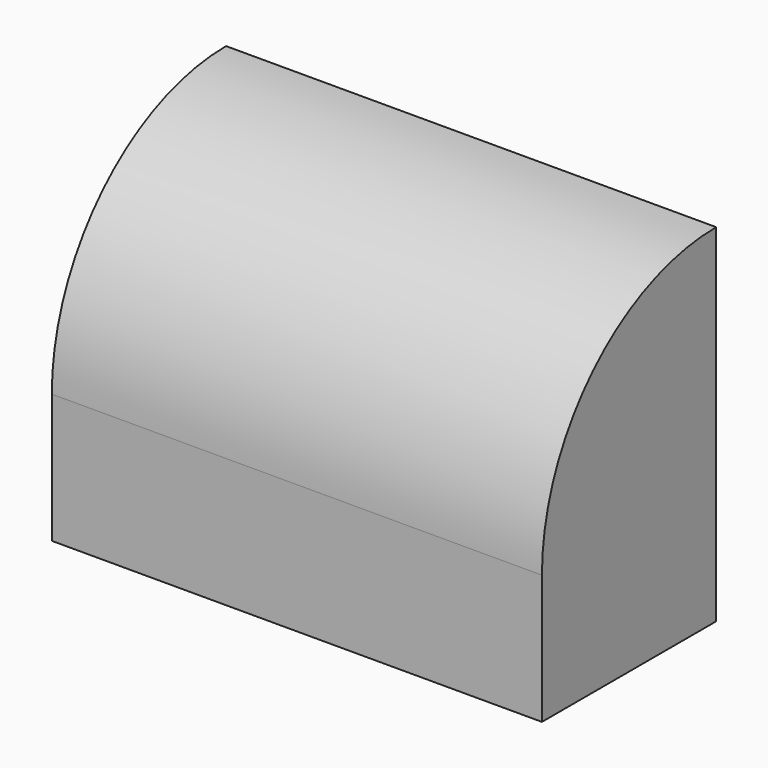
from build123d import *

# Parameters (mm, degrees)
F0_W     = 57.15
F0_H     = 40.463867586
F1_DEPTH = 25.4
F2_R     = 25.39999


# Not quite as in the source:
# - a fillet or chamfer is up to 0.001 mm smaller than in the source, because OpenCascade refuses the exact size


with BuildPart() as f1:
    # F0 (on Front) → F1 (new body)
    with BuildSketch(Plane.XZ):
        with Locations((-28.575, 20.231933793)):
            Rectangle(F0_W, F0_H)
    extrude(amount=F1_DEPTH)

    # F2 (radius 25.4 in the source; OpenCascade refuses exactly that, so slightly less here)
    f2_edges = [f1.edges().sort_by_distance(p)[0] for p in [
        (-28.575, -25.4, 40.463868),
    ]]
    fillet(f2_edges, radius=F2_R)


solid = f1.part
